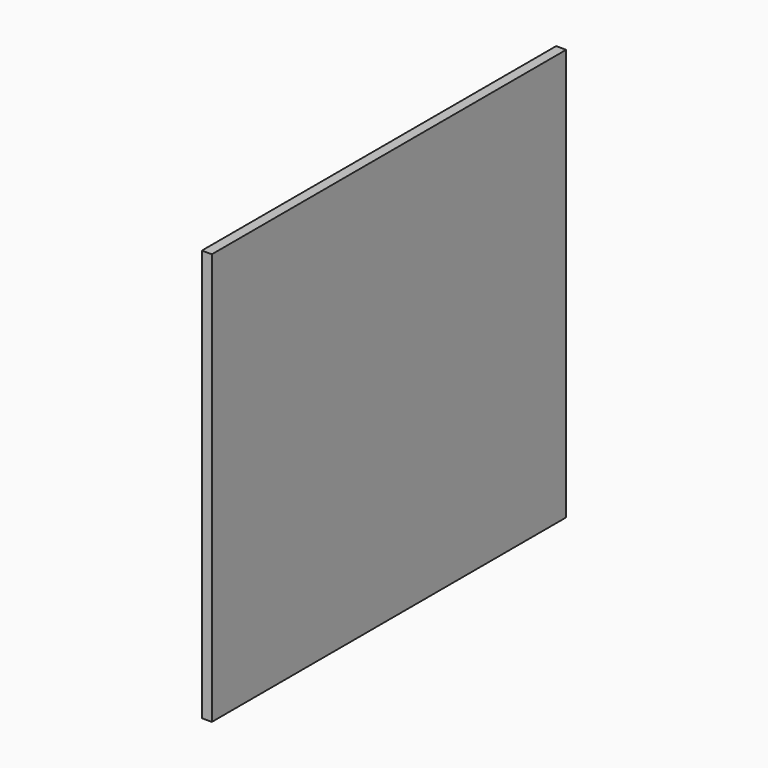
from build123d import *

# Parameters (mm, degrees)
F0_W          = 176.839619875
F0_H          = 164.3879562616
F1_DEPTH      = 2
F1_DEPTH_BACK = 2


# Not quite as in the source:
# - the program builds the solid bodies; features that only make, move or delete a surface that nothing else refers to are left out


with BuildPart() as f1:
    # F0 (on Right) → F1 (new body, two sides)
    with BuildSketch(Plane.YZ) as f1_sk:
        with Locations((2.6164352894, 0)):
            Rectangle(F0_W, F0_H)
    extrude(amount=F1_DEPTH)
    extrude(f1_sk.sketch, amount=-F1_DEPTH_BACK)


solid = f1.part
